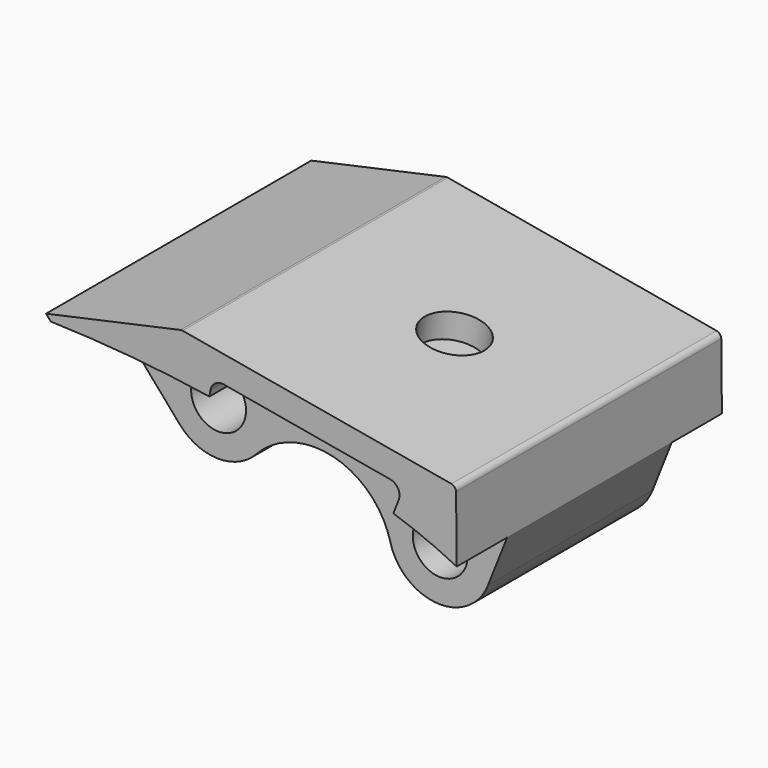
from build123d import *

# Parameters (mm, degrees)
F0_R     = 2.4
F1_DEPTH = 9
F2_DEPTH = 14.5
F3_R     = 0.5
F4_R     = 2.65
F5_DEPTH = 3


# Not quite as in the source:
# - two fillets or chamfers of one size are made in one step


with BuildPart() as f1:
    # F0 (on Front) → F1 (new body, symmetric)
    with BuildSketch(Plane.XZ):
        with BuildLine():
            Line((-19.2344364101, -14.475), (-12.351193111, -22.3932656305))
            ThreePointArc((-12.351193111, -22.3932656305), (-9.0297827018, -23.9403785735), (-5.6587929287, -22.5044978281))
            ThreePointArc((-5.6587929287, -22.5044978281), (1.0891796651, -20.5129837703), (6.0760796929, -25.4760564557))
            ThreePointArc((6.0760796929, -25.4760564557), (10.1567684842, -28.8420423371), (14.6192295456, -26.0015629336))
            Line((14.6192295456, -26.0015629336), (16.2763282151, -21.8))
            ThreePointArc((16.2763282151, -21.8), (13.5478934476, -20.5465737293), (10.7331243144, -19.5013424519))
            ThreePointArc((10.7331243144, -19.5013424519), (10.0239485931, -19.2751816233), (9.3106871937, -19.0622565188))
            ThreePointArc((9.3106871937, -19.0622565188), (2.0328204041, -17.1501268195), (-5.3587456661, -15.740043125))
            ThreePointArc((-5.3587456661, -15.740043125), (-12.2765411998, -14.887603878), (-19.2344364101, -14.475))
        make_face()
        with Locations((10.4330504183, -24.3505316455)):
            Circle(F0_R, mode=Mode.SUBTRACT)
        with Locations((-8.955, -19.441)):
            Circle(F0_R, mode=Mode.SUBTRACT)
        with BuildLine():
            Line((-19.6473476105, -14), (-19.2344364101, -14.475))
            ThreePointArc((-19.2344364101, -14.475), (-12.2765411998, -14.887603878), (-5.3587456661, -15.740043125))
            Line((-5.3587456661, -15.740043125), (-5.2650160599, -15.2084761138))
            ThreePointArc((-5.2650160599, -15.2084761138), (-4.8537847433, -14.5629722472), (-4.1065601293, -14.3973165385))
            Line((-4.1065601293, -14.3973165385), (10.4444975606, -16.9630606071))
            ThreePointArc((10.4444975606, -16.9630606071), (11.1434489978, -17.4594321695), (11.2011114112, -18.3147642019))
            Line((11.2011114112, -18.3147642019), (10.7331243144, -19.5013424519))
            ThreePointArc((10.7331243144, -19.5013424519), (13.5478934476, -20.5465737293), (16.2763282151, -21.8))
            Line((16.2763282151, -21.8), (16.2145160132, -15.6449893321))
            Line((16.2145160132, -15.6449893321), (-7.7940477934, -11.4116317649))
            Line((-7.7940477934, -11.4116317649), (-19.6473476105, -14))
        make_face()
    extrude(amount=F1_DEPTH, both=True)

    # F0 (on Front) → F2 (join, symmetric)
    with BuildSketch(Plane.XZ):
        with BuildLine():
            Line((-19.6473476105, -14), (-19.2344364101, -14.475))
            ThreePointArc((-19.2344364101, -14.475), (-12.2765411998, -14.887603878), (-5.3587456661, -15.740043125))
            Line((-5.3587456661, -15.740043125), (-5.2650160599, -15.2084761138))
            ThreePointArc((-5.2650160599, -15.2084761138), (-4.8537847433, -14.5629722472), (-4.1065601293, -14.3973165385))
            Line((-4.1065601293, -14.3973165385), (10.4444975606, -16.9630606071))
            ThreePointArc((10.4444975606, -16.9630606071), (11.1434489978, -17.4594321695), (11.2011114112, -18.3147642019))
            Line((11.2011114112, -18.3147642019), (10.7331243144, -19.5013424519))
            ThreePointArc((10.7331243144, -19.5013424519), (13.5478934476, -20.5465737293), (16.2763282151, -21.8))
            Line((16.2763282151, -21.8), (16.2145160132, -15.6449893321))
            Line((16.2145160132, -15.6449893321), (-7.7940477934, -11.4116317649))
            Line((-7.7940477934, -11.4116317649), (-19.6473476105, -14))
        make_face()
    extrude(amount=F2_DEPTH, both=True)

    # F3
    f3_edges = [f1.edges().sort_by_distance(p)[0] for p in [
        (-5.358746, 0, -15.740043),
        (10.733124, 0, -19.501342),
        (16.214516, 0, -15.644989),
        (-7.794048, 0, -11.411632),
    ]]
    fillet(f3_edges, radius=F3_R)

    # F4 (on face) → F5 (cut)
    with BuildSketch(Plane(origin=(-2.1865232639, 0, -12.4003896345), x_dir=(0.984807753, 0, -0.1736481777), z_dir=(0.1736481777, 0, 0.984807753))):
        with Locations((6.7739703659, 0)):
            Circle(F4_R)
    extrude(amount=-F5_DEPTH, mode=Mode.SUBTRACT)


solid = f1.part
